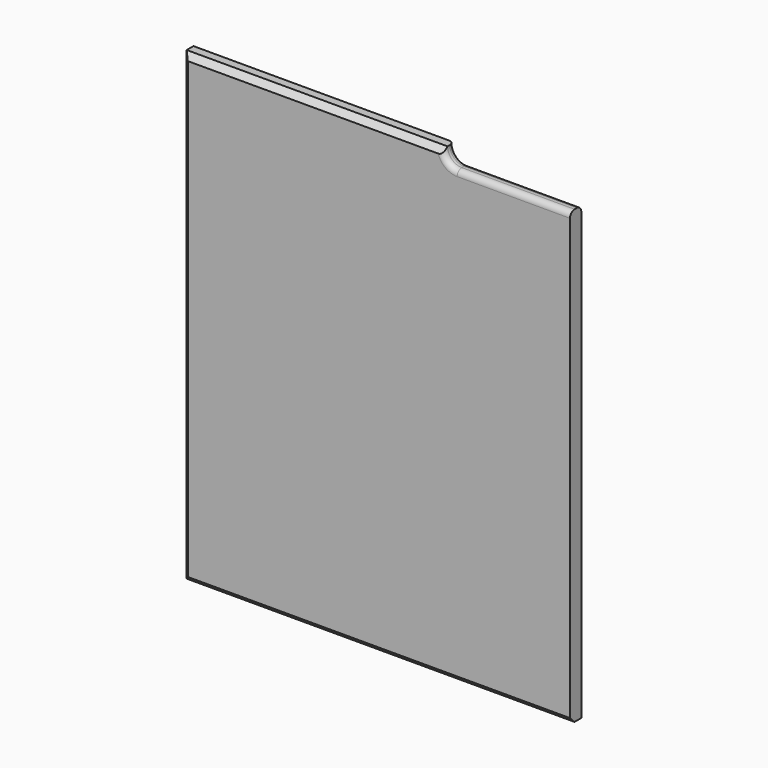
from build123d import *

# Parameters (mm, degrees)
F1_DEPTH    = 12.7
F2_R        = 5.08
F3_SIZE     = 5.08
F4_T1_DEPTH = 250.9182991577


# Not quite as in the source:
# - a fillet or chamfer that OpenCascade refuses, or shapes differently, is made with other operations: its cross-section is extruded or revolved along the edge and cut away or added


with BuildPart() as f1:
    # F0 (on Front) → F1 (new body)
    with BuildSketch(Plane.XZ):
        with BuildLine():
            Line((55.5559131622, 244.2450298561), (-179.3940868378, 244.2450298561))
            Line((-179.3940868378, 244.2450298561), (-179.3940868378, -174.8549701439))
            Line((-179.3940868378, -174.8549701439), (169.8559131622, -174.8549701439))
            Line((169.8559131622, -174.8549701439), (169.8559131622, 231.5450298561))
            Line((169.8559131622, 231.5450298561), (68.2559131622, 231.5450298561))
            ThreePointArc((68.2559131622, 231.5450298561), (59.2756570412, 235.264773735), (55.5559131622, 244.2450298561))
        make_face()
    extrude(amount=F1_DEPTH)

    # F2
    f2_edges = [f1.edges().sort_by_distance(p)[0] for p in [
        (119.055913, 0, 231.54503),
        (119.055913, -12.7, 231.54503),
        (59.275657, 0, 235.264774),
        (59.275657, -12.7, 235.264774),
    ]]
    fillet(f2_edges, radius=F2_R)

    # F3
    f3_edges = [f1.edges().sort_by_distance(p)[0] for p in [
        (-179.394087, -12.7, 34.69503),
        (-4.769087, -12.7, -174.85497),
    ]]
    chamfer(f3_edges, length=F3_SIZE)

    # F4: chamfer of 5.08 on 1 edges, made by hand

    # F4_s2 → F4_t1 (cut)
    with BuildSketch(Plane.YZ.offset(-187.3782364166)):
        Polygon((-7.62, 244.2450298561), (-12.7, 239.1650298561), (-12.7, 244.2450298561), align=None)
    extrude(amount=F4_T1_DEPTH, mode=Mode.SUBTRACT)


solid = f1.part
